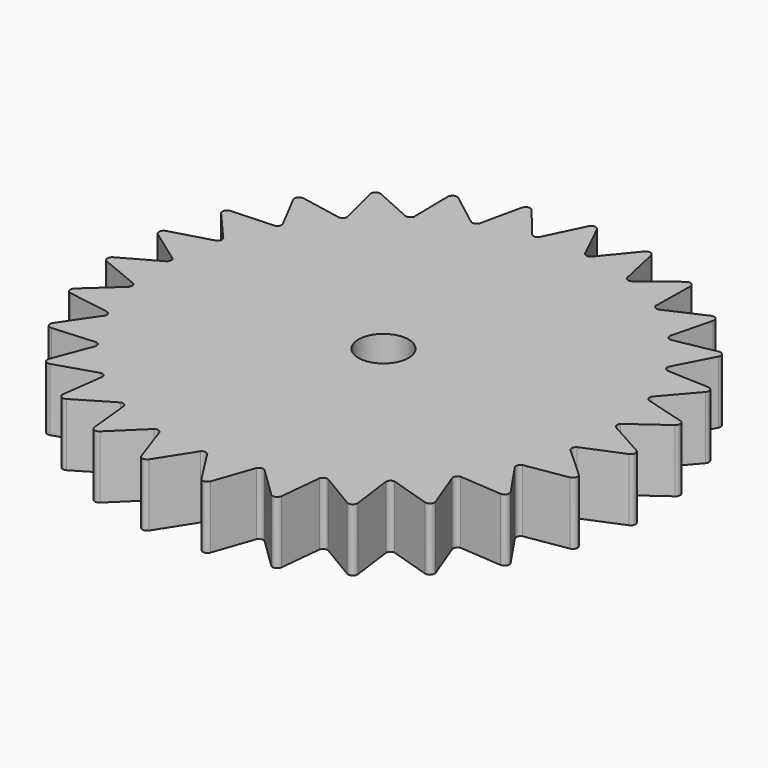
from build123d import *

# Parameters (mm, degrees)
F1_DEPTH = 4
F2_R     = 1.6
F3_DEPTH = 4.001


# Not quite as in the source:
# - ends of sketch curves that miss each other by under 0.0002 mm in the source are joined


with BuildPart() as f1:
    # F0 (on Top) → F1 (new body)
    with BuildSketch(Plane.XY):
        with BuildLine():
            ThreePointArc((1.9140106254, 14.2508572736), (1.6861265158, 14.1403198405), (1.4548574179, 14.2435879186))
            ThreePointArc((1.4548574179, 14.2435879186), (1.4306890387, 14.2754935862), (1.4109831428, 14.3103326425))
            Line((1.4109831428, 14.3103326425), (0.2558581901, 16.6921894723))
            ThreePointArc((0.2558581901, 16.6921894723), (0.1481039871, 16.8136670177), (-0.0071641706, 16.8612018631))
            ThreePointArc((-0.0071641706, 16.8612018631), (-0.1706127192, 16.817202235), (-0.2842271711, 16.6917305187))
            Line((-0.2842271711, 16.6917305187), (-1.4664410979, 14.2434227482))
            ThreePointArc((-1.4664410979, 14.2434227482), (-1.6902437576, 14.1388197245), (-1.916663057, 14.237631282))
            Line((-1.916663057, 14.237631282), (-3.6000092117, 16.3013673957))
            ThreePointArc((-3.6000092117, 16.3013673957), (-3.9019049125, 16.4036015506), (-4.125434594, 16.1763850942))
            Line((-4.125434594, 16.1763850942), (-4.7109828334, 13.5226488797))
            ThreePointArc((-4.7109828334, 13.5226488797), (-4.9015400565, 13.3688823231), (-5.1432019185, 13.4083253663))
            Line((-5.1432019185, 13.4083253663), (-7.2618513891, 15.0319710101))
            ThreePointArc((-7.2618513891, 15.0319710101), (-7.579185331, 15.0618374778), (-7.7442986009, 14.7892013747))
            Line((-7.7442986009, 14.7892013747), (-7.702174618, 12.0732144933))
            ThreePointArc((-7.702174618, 12.0732144933), (-7.8496947229, 11.8796668128), (-8.0921885063, 11.8591814286))
            Line((-8.0921885063, 11.8591814286), (-10.532310636, 12.9524153773))
            ThreePointArc((-10.532310636, 12.9524153773), (-10.8479798704, 12.9083044823), (-10.9457778263, 12.604942658))
            Line((-10.9457778263, 12.604942658), (-10.2788390418, 9.9731081586))
            ThreePointArc((-10.2788390418, 9.9731081586), (-10.375659889, 9.7510858631), (-10.6049250215, 9.6729470431))
            Line((-10.6049250215, 9.6729470431), (-13.2351231204, 10.1747796938))
            ThreePointArc((-13.2351231204, 10.1747796938), (-13.5321144192, 10.0590688256), (-13.5573261675, 9.7413311912))
            Line((-13.5573261675, 9.7413311912), (-12.3021100194, 7.3353788314))
            ThreePointArc((-12.3021100194, 7.3353788314), (-12.3432937572, 7.097610167), (-12.5462575743, 6.967089184))
            Line((-12.5462575743, 6.967089184), (-15.2246187544, 6.8487666996))
            ThreePointArc((-15.2246187544, 6.8487666996), (-15.4869255508, 6.6676921814), (-15.4381922857, 6.3527034427))
            Line((-15.4381922857, 6.3527034427), (-13.6629152877, 4.3020497532))
            ThreePointArc((-13.6629152877, 4.3020497532), (-13.6465657396, 4.062029571), (-13.8118007442, 3.8871742342))
            Line((-13.8118007442, 3.8871742342), (-16.3935721919, 3.153634337))
            ThreePointArc((-16.3935721919, 3.153634337), (-16.6070572662, 2.9169553146), (-16.4870055032, 2.621692024))
            Line((-16.4870055032, 2.621692024), (-14.2878546387, 1.0364711274))
            ThreePointArc((-14.2878546387, 1.0364711274), (-14.2152379851, 0.8077409694), (-14.3335516124, 0.5989526815))
            Line((-14.3335516124, 0.5989526815), (-16.6789818187, -0.7114654884))
            ThreePointArc((-16.6789818187, -0.7114654884), (-16.832139234, -0.9909930232), (-16.6472392521, -1.2506174313))
            Line((-16.6472392521, -1.2506174313), (-14.1431571391, -2.2854765977))
            ThreePointArc((-14.1431571391, -2.2854765977), (-14.0186393167, -2.4900607643), (-14.0835502146, -2.7205948066))
            Line((-14.0835502146, -2.7205948066), (-16.0654652706, -4.5382203487))
            ThreePointArc((-16.0654652706, -4.5382203487), (-16.1500404943, -4.8455310516), (-15.9102576154, -5.0555239268))
            Line((-15.9102576154, -5.0555239268), (-13.2365040498, -5.4848550701))
            ThreePointArc((-13.2365040498, -5.4848550701), (-13.0673141606, -5.6538228156), (-13.0753841374, -5.8928002059))
            Line((-13.0753841374, -5.8928002059), (-14.5860884781, -8.1203844463))
            ThreePointArc((-14.5860884781, -8.1203844463), (-14.5975232656, -8.4389155785), (-14.3157807663, -8.5879591986))
            Line((-14.3157807663, -8.5879591986), (-11.6166191171, -8.3893058066))
            ThreePointArc((-11.6166191171, -8.3893058066), (-11.4124537807, -8.5131996233), (-11.3634554587, -8.746935215))
            Line((-11.3634554587, -8.746935215), (-12.3205835531, -11.2648943843))
            ThreePointArc((-12.3205835531, -11.2648943843), (-12.258261618, -11.5774784738), (-11.9497442197, -11.6575400221))
            Line((-11.9497442197, -11.6575400221), (-9.3706481648, -10.8423342647))
            ThreePointArc((-9.3706481648, -10.8423342647), (-9.143139116, -10.914229028), (-9.0400495076, -11.1294074585))
            Line((-9.0400495076, -11.1294074585), (-9.3910515674, -13.8022744624))
            ThreePointArc((-9.3910515674, -13.8022744624), (-9.2583317968, -14.0920645572), (-8.9396672739, -14.0988290571))
            Line((-8.9396672739, -14.0988290571), (-6.6194690015, -12.711740107))
            ThreePointArc((-6.6194690015, -12.711740107), (-6.3815431901, -12.7276255469), (-6.2303634454, -12.912031956))
            Line((-6.2303634454, -12.912031956), (-5.955381825, -15.5957706951))
            ThreePointArc((-5.955381825, -15.5957706951), (-5.7594172495, -15.8471483428), (-5.4477802634, -15.7802512165))
            Line((-5.4477802634, -15.7802512165), (-3.5111841497, -13.8967395131))
            ThreePointArc((-3.5111841497, -13.8967395131), (-3.2763512695, -13.8557442651), (-3.0857625615, -13.9989330789))
            Line((-3.0857625615, -13.9989330789), (-2.1987423004, -16.54872127))
            ThreePointArc((-2.1987423004, -16.54872127), (-1.9500945765, -16.7481382853), (-1.6622810343, -16.6111850031))
            Line((-1.6622810343, -16.6111850031), (-0.2131467972, -14.3333958211))
            ThreePointArc((-0.2131467972, -14.3333958211), (0.005246929, -14.2378403367), (0.2243723928, -14.331705673))
            Line((0.2243723928, -14.331705673), (1.6764001268, -16.6097662074))
            ThreePointArc((1.6764001268, -16.6097662074), (1.9643299452, -16.746474862), (2.2128081189, -16.546846623))
            Line((2.2128081189, -16.546846623), (3.0970506062, -13.9980658779))
            ThreePointArc((3.0970506062, -13.9980658779), (3.286561705, -13.8533408388), (3.521767647, -13.8925576515))
            Line((3.521767647, -13.8925576515), (5.4611917751, -15.775615445))
            ThreePointArc((5.4611917751, -15.775615445), (5.7728854965, -15.8422477244), (5.9686363857, -15.5907036409))
            Line((5.9686363857, -15.5907036409), (6.2411397895, -12.9086763338))
            ThreePointArc((6.2411397895, -12.9086763338), (6.3909195318, -12.7229527682), (6.6288572495, -12.7052650163))
            Line((6.6288572495, -12.7052650163), (8.9516484854, -14.0912261582))
            ThreePointArc((8.9516484854, -14.0912261582), (9.2703071449, -14.0841908662), (9.4027806099, -13.7942880935))
            Line((9.4027806099, -13.7942880935), (9.0497770711, -11.1237609685))
            ThreePointArc((9.0497770711, -11.1237609685), (9.1511783498, -10.9075475026), (9.3783451778, -10.8338880535))
            Line((9.3783451778, -10.8338880535), (11.9596494988, -11.6473797597))
            ThreePointArc((11.9596494988, -11.6473797597), (12.268098751, -11.5670560686), (12.3301550361, -11.2544191321))
            Line((12.3301550361, -11.2544191321), (11.3716636637, -8.7393106928))
            ThreePointArc((11.3716636637, -8.7393106928), (11.4187295037, -8.5048818109), (11.6222137202, -8.3793180118))
            Line((11.6222137202, -8.3793180118), (14.3230763647, -8.5757891676))
            ThreePointArc((14.3230763647, -8.5757891676), (14.604692108, -8.4265061824), (14.5929866434, -8.1079848822))
            Line((14.5929866434, -8.1079848822), (13.0816946487, -5.8836056031))
            ThreePointArc((13.0816946487, -5.8836056031), (13.0715015116, -5.644332005), (13.2396929757, -5.4738404035))
            Line((13.2396929757, -5.4738404035), (15.9145504354, -5.0420000401))
            ThreePointArc((15.9145504354, -5.0420000401), (16.15415478, -4.8318034782), (16.0693184405, -4.5245647566))
            Line((16.0693184405, -4.5245647566), (14.0876977194, -2.7103070117))
            ThreePointArc((14.0876977194, -2.7103070117), (14.0205346934, -2.4799248131), (14.1437623045, -2.2740078751))
            Line((14.1437623045, -2.2740078751), (16.648298033, -1.2364685688))
            ThreePointArc((16.648298033, -1.2364685688), (16.8329773247, -0.9766871303), (16.6795824278, -0.6972898464))
            Line((16.6795824278, -0.6972898464), (14.335398798, 0.6098192161))
            ThreePointArc((14.335398798, 0.6098192161), (14.2147728105, 0.8179597828), (14.2858336525, 1.0477933771))
            Line((14.2858336525, 1.0477933771), (16.4847732853, 2.6357032988))
            ThreePointArc((16.4847732853, 2.6357032988), (16.6045740963, 2.9310685003), (16.3908879741, 3.1675660221))
            Line((16.3908879741, 3.1675660221), (13.8113473036, 3.8981036809))
            ThreePointArc((13.8113473036, 3.8981036809), (13.6438142546, 4.0717671277), (13.6583646175, 4.3126293336))
            Line((13.6583646175, 4.3126293336), (15.4327894801, 6.3658219818))
            ThreePointArc((15.4327894801, 6.3658219818), (15.4812550566, 6.6808520192), (15.2187944815, 6.8617035691))
            Line((15.2187944815, 6.8617035691), (12.5436443132, 6.9776065604))
            ThreePointArc((12.5436443132, 6.9776065604), (12.3384761371, 7.1063341886), (12.2952606451, 7.3446558284))
            Line((12.2952606451, 7.3446558284), (13.5490440665, 9.7528499611))
            ThreePointArc((13.5490440665, 9.7528499611), (13.5235623203, 10.0705660564), (13.2264728, 10.1860245057))
            Line((13.2264728, 10.1860245057), (10.6004372903, 9.6826728997))
            ThreePointArc((10.6004372903, 9.6826728997), (10.3691452759, 9.7583299946), (10.2700448298, 9.9805890632))
            Line((10.2700448298, 9.9805890632), (10.9350629039, 12.6142408462))
            ThreePointArc((10.9350629039, 12.6142408462), (10.8370071926, 12.9175194542), (10.5213005877, 12.961362084))
            Line((10.5213005877, 12.961362084), (8.0862749191, 11.8679259428))
            ThreePointArc((8.0862749191, 11.8679259428), (7.8420206158, 11.8850667554), (7.6918940409, 12.0784988717))
            Line((7.6918940409, 12.0784988717), (7.7317284499, 14.7957778483))
            ThreePointArc((7.7317284499, 14.7957778483), (7.566383559, 15.0682735431), (7.2490751116, 15.0381374223))
            Line((7.2490751116, 15.0381374223), (5.1365969535, 13.4163699229))
            ThreePointArc((5.1365969535, 13.4163699229), (4.8935343549, 13.3722272394), (4.6997550083, 13.5254511546))
            Line((4.6997550083, 13.5254511546), (4.1116867961, 16.1798854092))
            ThreePointArc((4.1116867961, 16.1798854092), (3.8879641114, 16.4069118327), (3.5861553961, 16.3044211699))
            Line((3.5861553961, 16.3044211699), (1.9140106254, 14.2508572736))
        make_face()
    extrude(amount=F1_DEPTH)

    # F2 (on face) → F3 (cut, through all)
    with BuildSketch(Plane.XY.offset(4)):
        Circle(F2_R)
    extrude(amount=-F3_DEPTH, mode=Mode.SUBTRACT)


solid = f1.part
